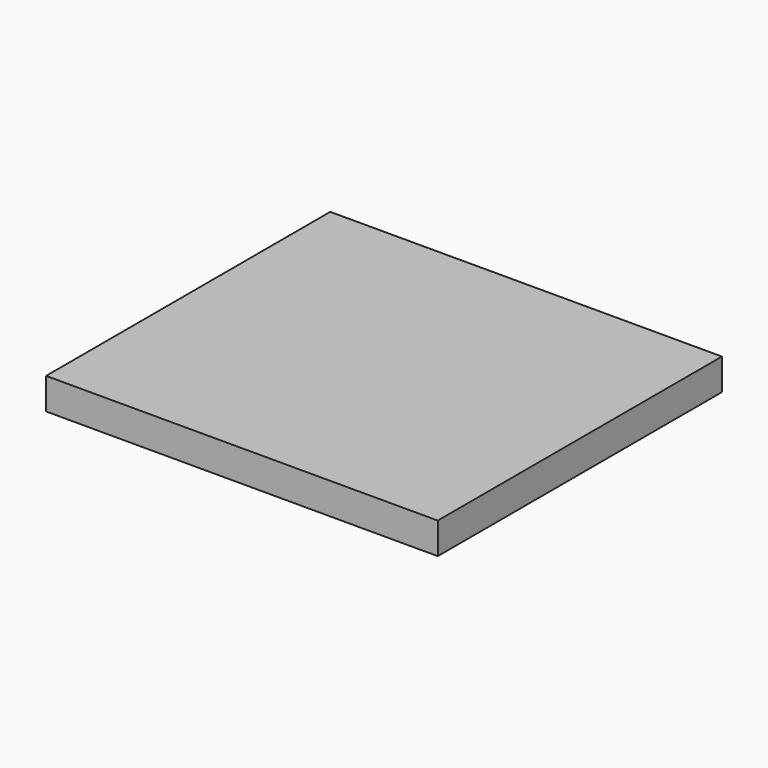
from build123d import *

# Parameters (mm, degrees)
F0_R     = 21.59
F1_DEPTH = 3.81
F2_W     = 47.6150820366
F2_H     = 43.18
F3_DEPTH = 3.81


# Not quite as in the source:
# - a feature of the source that left no trace in its solid (it failed there, or was rolled back) is left out


with BuildPart() as f1:
    # F0 (on Top) → F1 (new body)
    with BuildSketch(Plane.XY):
        Circle(F0_R)
    extrude(amount=F1_DEPTH)


with BuildPart() as f3:
    # F2 (on face) → F3 (new body)
    with BuildSketch(Plane(origin=(0, 0, 0), x_dir=(1, 0, 0), z_dir=(0, 0, -1))):
        Rectangle(F2_W, F2_H)
    extrude(amount=-F3_DEPTH)


solid = Compound([f1.part, f3.part])
